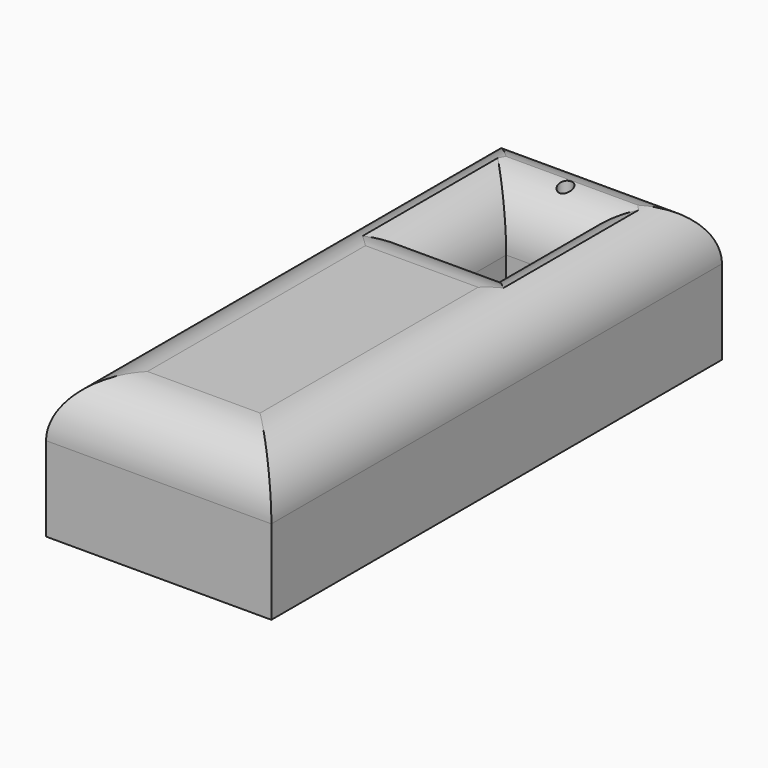
from build123d import *

# Parameters (mm, degrees)
F0_W         = 20.32
F0_H         = 50.8
F1_DEPTH     = 12.7
F2_W         = 15.24
F2_H         = 45.72
F3_DEPTH     = 5.08
F4_W         = 3.2004
F4_H         = 3.5052
F5_DEPTH     = 2.54
F6_W         = 5.08
F6_H         = 7.62
F7_DEPTH     = 25.4
F8_T1_DEPTH  = 76.2
F8_T3_DEPTH  = 45.72
F8_T5_DEPTH  = 7.62
F8_T7_DEPTH  = 5.08
F8_T13_DEPTH = 20.32
F8_T17_DEPTH = 17.78
F8_T24_DEPTH = 20.32
F8_T28_DEPTH = 17.78
F8_T35_DEPTH = 17.78
F8_T39_DEPTH = 20.32
F8_T46_DEPTH = 20.32
F8_T50_DEPTH = 17.78
F9_R         = 0.635
F10_DEPTH    = 25.4


# Not quite as in the source:
# - a fillet or chamfer that OpenCascade refuses, or shapes differently, is made with other operations: its cross-section is extruded or revolved along the edge and cut away or added


with BuildPart() as f1:
    # F0 (on Top) → F1 (new body)
    with BuildSketch(Plane.XY):
        Rectangle(F0_W, F0_H)
    extrude(amount=F1_DEPTH)

    # F2 (on Top) → F3 (cut)
    with BuildSketch(Plane.XY):
        Rectangle(F2_W, F2_H)
    extrude(amount=F3_DEPTH, mode=Mode.SUBTRACT)

    # F4 (on face) → F5 (cut)
    with BuildSketch(Plane(origin=(0, 0, 5.08), x_dir=(1, 0, 0), z_dir=(0, 0, -1))):
        with Locations((0, -20.5359)):
            Rectangle(F4_W, F4_H)
    extrude(amount=-F5_DEPTH, mode=Mode.SUBTRACT)

    # F6 (on Top) → F7 (cut)
    with BuildSketch(Plane.XY):
        with Locations((0, 13.1445)):
            Rectangle(F6_W, F6_H)
    extrude(amount=F7_DEPTH, mode=Mode.SUBTRACT)

    # F8: fillet of radius 5.08 on 8 edges, made by hand

    # F8_s2 → F8_t1 (cut)
    with BuildSketch(Plane.XZ.offset(-38.1)):
        with BuildLine():
            ThreePointArc((10.16, 7.62), (8.6721024484, 11.2121024484), (5.08, 12.7))
            Line((5.08, 12.7), (10.16, 12.7))
            Line((10.16, 12.7), (10.16, 7.62))
        make_face()
        with BuildLine():
            ThreePointArc((-5.08, 12.7), (-8.6721024484, 11.2121024484), (-10.16, 7.62))
            Line((-10.16, 7.62), (-10.16, 12.7))
            Line((-10.16, 12.7), (-5.08, 12.7))
        make_face()
    extrude(amount=F8_T1_DEPTH, mode=Mode.SUBTRACT)

    # F8_s4 → F8_t3 (cut)
    with BuildSketch(Plane.YZ.offset(-22.86)):
        with BuildLine():
            ThreePointArc((-25.4, 7.62), (-23.9121024484, 11.2121024484), (-20.32, 12.7))
            Line((-20.32, 12.7), (-25.4, 12.7))
            Line((-25.4, 12.7), (-25.4, 7.62))
        make_face()
        with BuildLine():
            ThreePointArc((25.4, 7.62), (23.9121024484, 11.2121024484), (20.32, 12.7))
            Line((20.32, 12.7), (25.4, 12.7))
            Line((25.4, 12.7), (25.4, 7.62))
        make_face()
    extrude(amount=F8_T3_DEPTH, mode=Mode.SUBTRACT)

    # F8_s6 → F8_t5 (cut)
    with BuildSketch(Plane.XZ.offset(-16.9545)):
        with BuildLine():
            ThreePointArc((7.62, 12.7), (4.0278975516, 11.2121024484), (2.54, 7.62))
            Line((2.54, 7.62), (2.54, 12.7))
            Line((2.54, 12.7), (7.62, 12.7))
        make_face()
        with BuildLine():
            ThreePointArc((-7.62, 12.7), (-4.0278975516, 11.2121024484), (-2.54, 7.62))
            Line((-2.54, 7.62), (-2.54, 12.7))
            Line((-2.54, 12.7), (-7.62, 12.7))
        make_face()
    extrude(amount=F8_T5_DEPTH, mode=Mode.SUBTRACT)

    # F8_s8 → F8_t7 (cut)
    with BuildSketch(Plane.YZ.offset(-2.54)):
        with BuildLine():
            ThreePointArc((22.0345, 12.7), (18.4423975516, 11.2121024484), (16.9545, 7.62))
            Line((16.9545, 7.62), (16.9545, 12.7))
            Line((16.9545, 12.7), (22.0345, 12.7))
        make_face()
        with BuildLine():
            ThreePointArc((4.2545, 12.7), (7.8466024484, 11.2121024484), (9.3345, 7.62))
            Line((9.3345, 7.62), (9.3345, 12.7))
            Line((9.3345, 12.7), (4.2545, 12.7))
        make_face()
    extrude(amount=F8_T7_DEPTH, mode=Mode.SUBTRACT)


with BuildPart() as f8_tool11:
    # F8_s12 → F8_t13 (new body)
    with BuildSketch(Plane.XZ.offset(-29.6545)):
        with BuildLine():
            ThreePointArc((7.62, 12.7), (4.0278975516, 11.2121024484), (2.54, 7.62))
            Line((2.54, 7.62), (2.54, 12.7))
            Line((2.54, 12.7), (7.62, 12.7))
        make_face()
    extrude(amount=F8_T13_DEPTH)

    split(bisect_by=Plane.XZ.offset(-16.9545), keep=Keep.BOTTOM)


with BuildPart() as f8_tool15:
    # F8_s16 → F8_t17 (new body)
    with BuildSketch(Plane.YZ.offset(-2.54)):
        with BuildLine():
            ThreePointArc((22.0345, 12.7), (18.4423975516, 11.2121024484), (16.9545, 7.62))
            Line((16.9545, 7.62), (16.9545, 12.7))
            Line((16.9545, 12.7), (22.0345, 12.7))
        make_face()
    extrude(amount=F8_T17_DEPTH)

    split(bisect_by=Plane.YZ.offset(2.54), keep=Keep.TOP)


with BuildPart() as f8_tool11_1:
    add(f8_tool11.part)

    # F8_t19: intersect F8_tool15
    add(f8_tool15.part, mode=Mode.INTERSECT)


with BuildPart() as f1_1:
    add(f1.part)

    # F8_t9: cut F8_tool11
    add(f8_tool11_1.part, mode=Mode.SUBTRACT)


with BuildPart() as f8_tool22:
    # F8_s23 → F8_t24 (new body)
    with BuildSketch(Plane.XZ.offset(-16.9545)):
        with BuildLine():
            ThreePointArc((7.62, 12.7), (4.0278975516, 11.2121024484), (2.54, 7.62))
            Line((2.54, 7.62), (2.54, 12.7))
            Line((2.54, 12.7), (7.62, 12.7))
        make_face()
    extrude(amount=F8_T24_DEPTH)

    split(bisect_by=Plane.XZ.offset(-9.3345), keep=Keep.TOP)


with BuildPart() as f8_tool26:
    # F8_s27 → F8_t28 (new body)
    with BuildSketch(Plane.YZ.offset(15.24)):
        with BuildLine():
            ThreePointArc((4.2545, 12.7), (7.8466024484, 11.2121024484), (9.3345, 7.62))
            Line((9.3345, 7.62), (9.3345, 12.7))
            Line((9.3345, 12.7), (4.2545, 12.7))
        make_face()
    extrude(amount=-F8_T28_DEPTH)

    split(bisect_by=Plane.YZ.offset(2.54), keep=Keep.TOP)


with BuildPart() as f8_tool22_1:
    add(f8_tool22.part)

    # F8_t30: intersect F8_tool26
    add(f8_tool26.part, mode=Mode.INTERSECT)


with BuildPart() as f1_2:
    add(f1_1.part)

    # F8_t20: cut F8_tool22
    add(f8_tool22_1.part, mode=Mode.SUBTRACT)


with BuildPart() as f8_tool33:
    # F8_s34 → F8_t35 (new body)
    with BuildSketch(Plane.YZ.offset(-15.24)):
        with BuildLine():
            ThreePointArc((22.0345, 12.7), (18.4423975516, 11.2121024484), (16.9545, 7.62))
            Line((16.9545, 7.62), (16.9545, 12.7))
            Line((16.9545, 12.7), (22.0345, 12.7))
        make_face()
    extrude(amount=F8_T35_DEPTH)

    split(bisect_by=Plane.YZ.offset(-2.54), keep=Keep.BOTTOM)


with BuildPart() as f8_tool37:
    # F8_s38 → F8_t39 (new body)
    with BuildSketch(Plane.XZ.offset(-9.3345)):
        with BuildLine():
            ThreePointArc((-7.62, 12.7), (-4.0278975516, 11.2121024484), (-2.54, 7.62))
            Line((-2.54, 7.62), (-2.54, 12.7))
            Line((-2.54, 12.7), (-7.62, 12.7))
        make_face()
    extrude(amount=-F8_T39_DEPTH)

    split(bisect_by=Plane.XZ.offset(-16.9545), keep=Keep.BOTTOM)


with BuildPart() as f8_tool33_1:
    add(f8_tool33.part)

    # F8_t41: intersect F8_tool37
    add(f8_tool37.part, mode=Mode.INTERSECT)


with BuildPart() as f1_3:
    add(f1_2.part)

    # F8_t31: cut F8_tool33
    add(f8_tool33_1.part, mode=Mode.SUBTRACT)


with BuildPart() as f8_tool44:
    # F8_s45 → F8_t46 (new body)
    with BuildSketch(Plane.XZ.offset(3.3655)):
        with BuildLine():
            ThreePointArc((-7.62, 12.7), (-4.0278975516, 11.2121024484), (-2.54, 7.62))
            Line((-2.54, 7.62), (-2.54, 12.7))
            Line((-2.54, 12.7), (-7.62, 12.7))
        make_face()
    extrude(amount=-F8_T46_DEPTH)

    split(bisect_by=Plane.XZ.offset(-9.3345), keep=Keep.TOP)


with BuildPart() as f8_tool48:
    # F8_s49 → F8_t50 (new body)
    with BuildSketch(Plane.YZ.offset(2.54)):
        with BuildLine():
            ThreePointArc((4.2545, 12.7), (7.8466024484, 11.2121024484), (9.3345, 7.62))
            Line((9.3345, 7.62), (9.3345, 12.7))
            Line((9.3345, 12.7), (4.2545, 12.7))
        make_face()
    extrude(amount=-F8_T50_DEPTH)

    split(bisect_by=Plane.YZ.offset(-2.54), keep=Keep.BOTTOM)


with BuildPart() as f8_tool44_1:
    add(f8_tool44.part)

    # F8_t52: intersect F8_tool48
    add(f8_tool48.part, mode=Mode.INTERSECT)


with BuildPart() as f1_4:
    add(f1_3.part)

    # F8_t42: cut F8_tool44
    add(f8_tool44_1.part, mode=Mode.SUBTRACT)

    # F9 (on face) → F10 (cut)
    with BuildSketch(Plane(origin=(0, 0, 7.62), x_dir=(1, 0, 0), z_dir=(0, 0, -1))):
        with Locations((0, -20.460145548)):
            Circle(F9_R)
    extrude(amount=-F10_DEPTH, mode=Mode.SUBTRACT)


solid = f1_4.part
